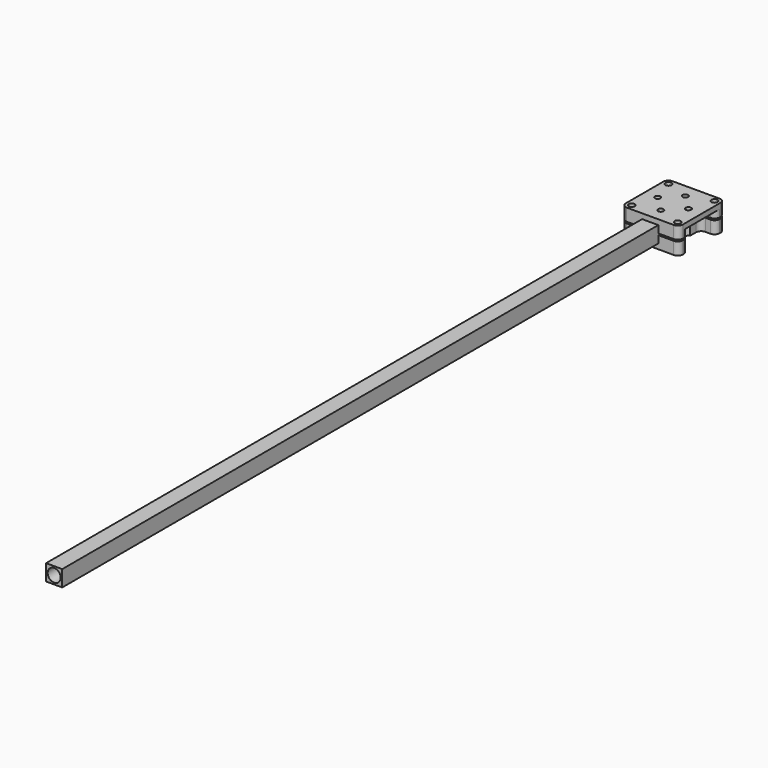
from build123d import *

# Parameters (mm, degrees)
F0_W      = 10
F0_H      = 10
F0_R      = 4
F1_DEPTH  = 250
F2_R      = 1.7
F2_R_2    = 1.89865
F3_DEPTH  = 3.175
F4_R      = 1.89865
F5_DEPTH  = 4.5
F7_R      = 1.89865
F8_DEPTH  = 4.5
F9_R      = 1.89865
F10_DEPTH = 3.175


with BuildPart() as f1:
    # F0 (on Front) → F1 (new body, symmetric)
    with BuildSketch(Plane.XZ):
        Rectangle(F0_W, F0_H)
        Circle(F0_R, mode=Mode.SUBTRACT)
    extrude(amount=F1_DEPTH, both=True)


with BuildPart() as f3:
    # F2 (on face) → F3 (new body)
    with BuildSketch(Plane.XY.offset(5)):
        with BuildLine():
            ThreePointArc((5, 216.060063796), (11.1747483193, 221.0253712962), (13.5, 228.6))
            ThreePointArc((13.5, 228.6), (11.1747483193, 236.1746287038), (5, 241.139936204))
            Line((5, 241.139936204), (5, 216.060063796))
        make_face()
        with Locations((9.5, 228.6)):
            Circle(F2_R, mode=Mode.SUBTRACT)
        with BuildLine():
            ThreePointArc((5, 241.139936204), (11.1747483193, 236.1746287038), (13.5, 228.6))
            ThreePointArc((13.5, 228.6), (11.1747483193, 221.0253712962), (5, 216.060063796))
            Line((5, 216.060063796), (5, 212.6922778186))
            ThreePointArc((5, 212.6922778186), (13.4430395558, 218.7338805754), (16.675, 228.6))
            ThreePointArc((16.675, 228.6), (13.4430395558, 238.4661194246), (5, 244.5077221814))
            Line((5, 244.5077221814), (5, 241.139936204))
        make_face()
        with BuildLine():
            Line((5, 216.060063796), (5, 241.139936204))
            ThreePointArc((5, 241.139936204), (0, 242.1), (-5, 241.139936204))
            Line((-5, 241.139936204), (-5, 216.060063796))
            ThreePointArc((-5, 216.060063796), (0, 215.1), (5, 216.060063796))
        make_face()
        with Locations((0, 219.1)):
            Circle(F2_R, mode=Mode.SUBTRACT)
        with Locations((0, 238.1)):
            Circle(F2_R, mode=Mode.SUBTRACT)
        with BuildLine():
            ThreePointArc((-5, 241.139936204), (0, 242.1), (5, 241.139936204))
            Line((5, 241.139936204), (5, 244.5077221814))
            ThreePointArc((5, 244.5077221814), (0, 245.275), (-5, 244.5077221814))
            Line((-5, 244.5077221814), (-5, 241.139936204))
        make_face()
        with BuildLine():
            Line((5, 212.6922778186), (5, 216.060063796))
            ThreePointArc((5, 216.060063796), (0, 215.1), (-5, 216.060063796))
            Line((-5, 216.060063796), (-5, 212.6922778186))
            ThreePointArc((-5, 212.6922778186), (0, 211.925), (5, 212.6922778186))
        make_face()
        with BuildLine():
            Line((-5, 216.060063796), (-5, 241.139936204))
            ThreePointArc((-5, 241.139936204), (-13.5, 228.6), (-5, 216.060063796))
        make_face()
        with Locations((-9.5, 228.6)):
            Circle(F2_R, mode=Mode.SUBTRACT)
        with BuildLine():
            ThreePointArc((-5, 216.060063796), (-13.5, 228.6), (-5, 241.139936204))
            Line((-5, 241.139936204), (-5, 244.5077221814))
            ThreePointArc((-5, 244.5077221814), (-16.675, 228.6), (-5, 212.6922778186))
            Line((-5, 212.6922778186), (-5, 216.060063796))
        make_face()
        with BuildLine():
            Line((5, 246.3), (5, 244.5077221814))
            ThreePointArc((5, 244.5077221814), (13.4430395558, 238.4661194246), (16.675, 228.6))
            ThreePointArc((16.675, 228.6), (13.4430395558, 218.7338805754), (5, 212.6922778186))
            Line((5, 212.6922778186), (5, 210.9))
            Line((5, 210.9), (14.525, 210.9))
            ThreePointArc((14.525, 210.9), (16.7700640303, 211.8299359697), (17.7, 214.075))
            Line((17.7, 214.075), (17.7, 243.125))
            ThreePointArc((17.7, 243.125), (16.7700640303, 245.3700640303), (14.525, 246.3))
            Line((14.525, 246.3), (5, 246.3))
        make_face()
        with Locations((14.21385, 214.38615)):
            Circle(F2_R_2, mode=Mode.SUBTRACT)
        with Locations((14.21385, 242.81385)):
            Circle(F2_R_2, mode=Mode.SUBTRACT)
        with BuildLine():
            ThreePointArc((-5, 244.5077221814), (0, 245.275), (5, 244.5077221814))
            Line((5, 244.5077221814), (5, 246.3))
            Line((5, 246.3), (-5, 246.3))
            Line((-5, 246.3), (-5, 244.5077221814))
        make_face()
        with BuildLine():
            Line((5, 210.9), (5, 212.6922778186))
            ThreePointArc((5, 212.6922778186), (0, 211.925), (-5, 212.6922778186))
            Line((-5, 212.6922778186), (-5, 210.9))
            Line((-5, 210.9), (5, 210.9))
        make_face()
        with BuildLine():
            ThreePointArc((-5, 212.6922778186), (-16.675, 228.6), (-5, 244.5077221814))
            Line((-5, 244.5077221814), (-5, 246.3))
            Line((-5, 246.3), (-14.525, 246.3))
            ThreePointArc((-14.525, 246.3), (-16.7700640303, 245.3700640303), (-17.7, 243.125))
            Line((-17.7, 243.125), (-17.7, 214.075))
            ThreePointArc((-17.7, 214.075), (-16.7700640303, 211.8299359697), (-14.525, 210.9))
            Line((-14.525, 210.9), (-5, 210.9))
            Line((-5, 210.9), (-5, 212.6922778186))
        make_face()
        with Locations((-14.21385, 214.38615)):
            Circle(F2_R_2, mode=Mode.SUBTRACT)
        with Locations((-14.21385, 242.81385)):
            Circle(F2_R_2, mode=Mode.SUBTRACT)
    extrude(amount=F3_DEPTH)

    # F4 (on face) → F5 (join)
    with BuildSketch(Plane(origin=(0, 0, 5), x_dir=(1, 0, 0), z_dir=(0, 0, -1))):
        with BuildLine():
            ThreePointArc((-17.7, -214.6973), (-16.7700640303, -216.9423640303), (-14.525, -217.8723))
            Line((-14.525, -217.8723), (-11.35, -217.8723))
            ThreePointArc((-11.35, -217.8723), (-9.1049359697, -218.8022359697), (-8.175, -221.0473))
            Line((-8.175, -221.0473), (-8.175, -225.6323620504))
            ThreePointArc((-8.175, -225.6323620504), (-6.25, -228.6), (-8.175, -231.5676379496))
            Line((-8.175, -231.5676379496), (-8.175, -236.1527))
            ThreePointArc((-8.175, -236.1527), (-9.1049359697, -238.3977640303), (-11.35, -239.3277))
            Line((-11.35, -239.3277), (-14.525, -239.3277))
            ThreePointArc((-14.525, -239.3277), (-16.7700640303, -240.2576359697), (-17.7, -242.5027))
            Line((-17.7, -242.5027), (-17.7, -243.125))
            ThreePointArc((-17.7, -243.125), (-16.7700640303, -245.3700640303), (-14.525, -246.3))
            Line((-14.525, -246.3), (-5, -246.3))
            Line((-5, -246.3), (-5, -210.9))
            Line((-5, -210.9), (-14.525, -210.9))
            ThreePointArc((-14.525, -210.9), (-16.7700640303, -211.8299359697), (-17.7, -214.075))
            Line((-17.7, -214.075), (-17.7, -214.6973))
        make_face()
        with Locations((-14.21385, -242.81385)):
            Circle(F4_R, mode=Mode.SUBTRACT)
        with Locations((-14.21385, -214.38615)):
            Circle(F4_R, mode=Mode.SUBTRACT)
        with BuildLine():
            Line((14.525, -210.9), (5, -210.9))
            Line((5, -210.9), (5, -246.3))
            Line((5, -246.3), (14.525, -246.3))
            ThreePointArc((14.525, -246.3), (16.7700640303, -245.3700640303), (17.7, -243.125))
            Line((17.7, -243.125), (17.7, -242.5027))
            ThreePointArc((17.7, -242.5027), (16.7700640303, -240.2576359697), (14.525, -239.3277))
            Line((14.525, -239.3277), (11.35, -239.3277))
            ThreePointArc((11.35, -239.3277), (9.1049359697, -238.3977640303), (8.175, -236.1527))
            Line((8.175, -236.1527), (8.175, -231.5676379496))
            ThreePointArc((8.175, -231.5676379496), (6.25, -228.6), (8.175, -225.6323620504))
            Line((8.175, -225.6323620504), (8.175, -221.0473))
            ThreePointArc((8.175, -221.0473), (9.1049359697, -218.8022359697), (11.35, -217.8723))
            Line((11.35, -217.8723), (14.525, -217.8723))
            ThreePointArc((14.525, -217.8723), (16.7700640303, -216.9423640303), (17.7, -214.6973))
            Line((17.7, -214.6973), (17.7, -214.075))
            ThreePointArc((17.7, -214.075), (16.7700640303, -211.8299359697), (14.525, -210.9))
        make_face()
        with Locations((14.21385, -242.81385)):
            Circle(F4_R, mode=Mode.SUBTRACT)
        with Locations((14.21385, -214.38615)):
            Circle(F4_R, mode=Mode.SUBTRACT)
    extrude(amount=F5_DEPTH)


with BuildPart() as f8:
    # F7 (on offset) → F8 (new body)
    with BuildSketch(Plane(origin=(0, 0, -0.5), x_dir=(1, 0, 0), z_dir=(0, 0, -1))):
        with BuildLine():
            Line((-5, -210.9), (-14.525, -210.9))
            ThreePointArc((-14.525, -210.9), (-16.7700640303, -211.8299359697), (-17.7, -214.075))
            Line((-17.7, -214.075), (-17.7, -214.6973))
            ThreePointArc((-17.7, -214.6973), (-16.7700640303, -216.9423640303), (-14.525, -217.8723))
            Line((-14.525, -217.8723), (-11.35, -217.8723))
            ThreePointArc((-11.35, -217.8723), (-9.1049359697, -218.8022359697), (-8.175, -221.0473))
            Line((-8.175, -221.0473), (-8.175, -225.6323620504))
            ThreePointArc((-8.175, -225.6323620504), (-6.25, -228.6), (-8.175, -231.5676379496))
            Line((-8.175, -231.5676379496), (-8.175, -236.1527))
            ThreePointArc((-8.175, -236.1527), (-9.1049359697, -238.3977640303), (-11.35, -239.3277))
            Line((-11.35, -239.3277), (-14.525, -239.3277))
            ThreePointArc((-14.525, -239.3277), (-16.7700640303, -240.2576359697), (-17.7, -242.5027))
            Line((-17.7, -242.5027), (-17.7, -243.125))
            ThreePointArc((-17.7, -243.125), (-16.7700640303, -245.3700640303), (-14.525, -246.3))
            Line((-14.525, -246.3), (-5, -246.3))
            Line((-5, -246.3), (-5, -210.9))
        make_face()
        with Locations((-14.21385, -242.81385)):
            Circle(F7_R, mode=Mode.SUBTRACT)
        with Locations((-14.21385, -214.38615)):
            Circle(F7_R, mode=Mode.SUBTRACT)
    extrude(amount=F8_DEPTH)



with BuildPart() as f8b:
    # F7 (on offset) → F8, piece 2 (new body)
    with BuildSketch(Plane(origin=(0, 0, -0.5), x_dir=(1, 0, 0), z_dir=(0, 0, -1))):
        with BuildLine():
            Line((5, -210.9), (5, -246.3))
            Line((5, -246.3), (14.525, -246.3))
            ThreePointArc((14.525, -246.3), (16.7700640303, -245.3700640303), (17.7, -243.125))
            Line((17.7, -243.125), (17.7, -242.5027))
            ThreePointArc((17.7, -242.5027), (16.7700640303, -240.2576359697), (14.525, -239.3277))
            Line((14.525, -239.3277), (11.35, -239.3277))
            ThreePointArc((11.35, -239.3277), (9.1049359697, -238.3977640303), (8.175, -236.1527))
            Line((8.175, -236.1527), (8.175, -231.5676379496))
            ThreePointArc((8.175, -231.5676379496), (6.25, -228.6), (8.175, -225.6323620504))
            Line((8.175, -225.6323620504), (8.175, -221.0473))
            ThreePointArc((8.175, -221.0473), (9.1049359697, -218.8022359697), (11.35, -217.8723))
            Line((11.35, -217.8723), (14.525, -217.8723))
            ThreePointArc((14.525, -217.8723), (16.7700640303, -216.9423640303), (17.7, -214.6973))
            Line((17.7, -214.6973), (17.7, -214.075))
            ThreePointArc((17.7, -214.075), (16.7700640303, -211.8299359697), (14.525, -210.9))
            Line((14.525, -210.9), (5, -210.9))
        make_face()
        with Locations((14.21385, -242.81385)):
            Circle(F7_R, mode=Mode.SUBTRACT)
        with Locations((14.21385, -214.38615)):
            Circle(F7_R, mode=Mode.SUBTRACT)
    extrude(amount=F8_DEPTH)


with BuildPart() as f8_1:
    add(f8.part)

    add(f8b.part)  # F10 merges F8b
    # F9 (on face) → F10 (join)
    with BuildSketch(Plane(origin=(0, 0, -5), x_dir=(1, 0, 0), z_dir=(0, 0, -1))):
        with BuildLine():
            Line((-5, -210.9), (-5, -246.3))
            Line((-5, -246.3), (5, -246.3))
            Line((5, -246.3), (14.525, -246.3))
            ThreePointArc((14.525, -246.3), (16.7700640303, -245.3700640303), (17.7, -243.125))
            Line((17.7, -243.125), (17.7, -242.5027))
            ThreePointArc((17.7, -242.5027), (16.7700640303, -240.2576359697), (14.525, -239.3277))
            Line((14.525, -239.3277), (11.35, -239.3277))
            ThreePointArc((11.35, -239.3277), (9.1049359697, -238.3977640303), (8.175, -236.1527))
            Line((8.175, -236.1527), (8.175, -231.5676379496))
            ThreePointArc((8.175, -231.5676379496), (6.25, -228.6), (8.175, -225.6323620504))
            Line((8.175, -225.6323620504), (8.175, -221.0473))
            ThreePointArc((8.175, -221.0473), (9.1049359697, -218.8022359697), (11.35, -217.8723))
            Line((11.35, -217.8723), (14.525, -217.8723))
            ThreePointArc((14.525, -217.8723), (16.7700640303, -216.9423640303), (17.7, -214.6973))
            Line((17.7, -214.6973), (17.7, -214.075))
            ThreePointArc((17.7, -214.075), (16.7700640303, -211.8299359697), (14.525, -210.9))
            Line((14.525, -210.9), (5, -210.9))
            Line((5, -210.9), (-5, -210.9))
        make_face()
        with Locations((14.21385, -242.81385)):
            Circle(F9_R, mode=Mode.SUBTRACT)
        with Locations((14.21385, -214.38615)):
            Circle(F9_R, mode=Mode.SUBTRACT)
        with BuildLine():
            Line((-14.525, -246.3), (-5, -246.3))
            Line((-5, -246.3), (-5, -210.9))
            Line((-5, -210.9), (-14.525, -210.9))
            ThreePointArc((-14.525, -210.9), (-16.7700640303, -211.8299359697), (-17.7, -214.075))
            Line((-17.7, -214.075), (-17.7, -214.6973))
            ThreePointArc((-17.7, -214.6973), (-16.7700640303, -216.9423640303), (-14.525, -217.8723))
            Line((-14.525, -217.8723), (-11.35, -217.8723))
            ThreePointArc((-11.35, -217.8723), (-9.1049359697, -218.8022359697), (-8.175, -221.0473))
            Line((-8.175, -221.0473), (-8.175, -225.6323620504))
            ThreePointArc((-8.175, -225.6323620504), (-6.25, -228.6), (-8.175, -231.5676379496))
            Line((-8.175, -231.5676379496), (-8.175, -236.1527))
            ThreePointArc((-8.175, -236.1527), (-9.1049359697, -238.3977640303), (-11.35, -239.3277))
            Line((-11.35, -239.3277), (-14.525, -239.3277))
            ThreePointArc((-14.525, -239.3277), (-16.7700640303, -240.2576359697), (-17.7, -242.5027))
            Line((-17.7, -242.5027), (-17.7, -243.125))
            ThreePointArc((-17.7, -243.125), (-16.7700640303, -245.3700640303), (-14.525, -246.3))
        make_face()
        with Locations((-14.21385, -242.81385)):
            Circle(F9_R, mode=Mode.SUBTRACT)
        with Locations((-14.21385, -214.38615)):
            Circle(F9_R, mode=Mode.SUBTRACT)
    extrude(amount=F10_DEPTH)


solid = Compound([f1.part, f3.part, f8_1.part])
